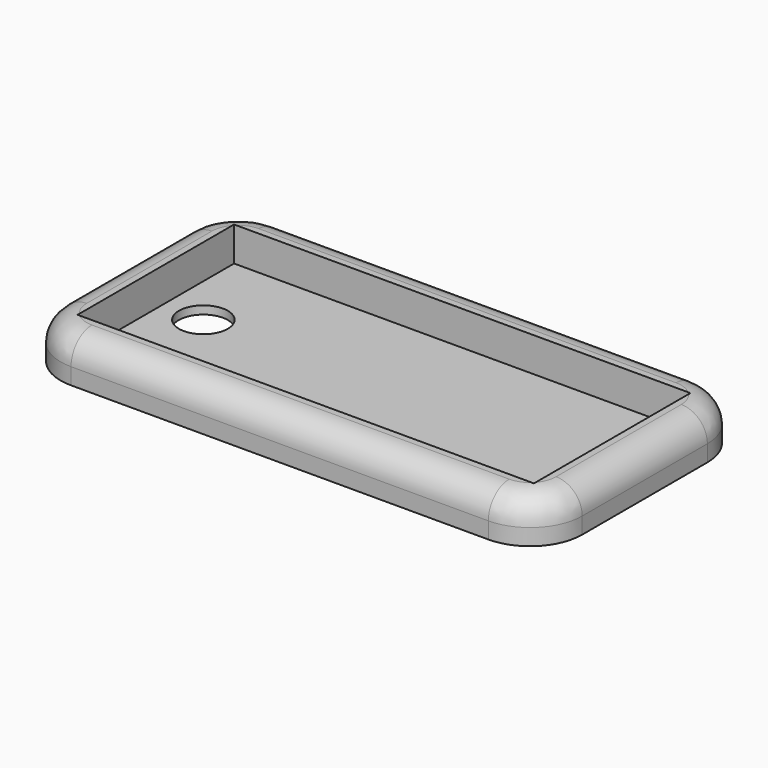
from build123d import *

# Parameters (mm, degrees)
F0_W         = 44.45
F0_H         = 19.05
F0_R         = 2.38125
F1_DEPTH     = 0.79375
F2_DEPTH     = 4.1402
F3_R         = 5.08
F4_T1_DEPTH  = 40.64
F4_T3_DEPTH  = 15.24
F4_T6_ANGLE  = 90
F4_T8_ANGLE  = 90
F4_T10_ANGLE = 90
F4_T12_ANGLE = 90


# Not quite as in the source:
# - a fillet or chamfer that OpenCascade refuses, or shapes differently, is made with other operations: its cross-section is extruded or revolved along the edge and cut away or added


with BuildPart() as f1:
    # F0 (on Top) → F1 (new body)
    with BuildSketch(Plane.XY):
        with Locations((25.4, 11.0452919405)):
            Rectangle(F0_W, F0_H)
        with Locations((7.14375, 11.8726459702)):
            Circle(F0_R, mode=Mode.SUBTRACT)
    extrude(amount=F1_DEPTH)

    # F0 (on Top) → F2 (join)
    with BuildSketch(Plane.XY):
        Polygon((0, 23.7452919405), (0, 0), (0, -1.6547080595), (50.8, -1.6547080595), (50.8, 23.7452919405), align=None)
        with Locations((25.4, 11.0452919405)):
            Rectangle(F0_W, F0_H, mode=Mode.SUBTRACT)
    extrude(amount=F2_DEPTH)

    # F3
    f3_edges = [f1.edges().sort_by_distance(p)[0] for p in [
        (50.8, -1.654708, 2.0701),
        (0, -1.654708, 2.0701),
        (50.8, 23.745292, 2.0701),
        (0, 23.745292, 2.0701),
    ]]
    fillet(f3_edges, radius=F3_R)

    # F4: fillet of radius 2.54 on 8 edges, made by hand

    # F4_s2 → F4_t1 (cut)
    with BuildSketch(Plane.YZ.offset(5.08)):
        with BuildLine():
            ThreePointArc((-1.6547080595, 1.6002), (-0.9107592837, 3.3962512242), (0.8852919405, 4.1402))
            Line((0.8852919405, 4.1402), (-1.6547080595, 4.1402))
            Line((-1.6547080595, 4.1402), (-1.6547080595, 1.6002))
        make_face()
        with BuildLine():
            ThreePointArc((23.7452919405, 1.6002), (23.0013431647, 3.3962512242), (21.2052919405, 4.1402))
            Line((21.2052919405, 4.1402), (23.7452919405, 4.1402))
            Line((23.7452919405, 4.1402), (23.7452919405, 1.6002))
        make_face()
    extrude(amount=F4_T1_DEPTH, mode=Mode.SUBTRACT)

    # F4_s4 → F4_t3 (cut)
    with BuildSketch(Plane.XZ.offset(-18.6652919405)):
        with BuildLine():
            ThreePointArc((0, 1.6002), (0.7439487758, 3.3962512242), (2.54, 4.1402))
            Line((2.54, 4.1402), (0, 4.1402))
            Line((0, 4.1402), (0, 1.6002))
        make_face()
        with BuildLine():
            ThreePointArc((50.8, 1.6002), (50.0560512242, 3.3962512242), (48.26, 4.1402))
            Line((48.26, 4.1402), (50.8, 4.1402))
            Line((50.8, 4.1402), (50.8, 1.6002))
        make_face()
    extrude(amount=F4_T3_DEPTH, mode=Mode.SUBTRACT)

    # F4_s5 → F4_t6 (revolve, cut)
    with BuildSketch(Plane.XZ.offset(-18.6652919405)):
        with BuildLine():
            ThreePointArc((0, 1.6002), (0.7439487758, 3.3962512242), (2.54, 4.1402))
            Line((2.54, 4.1402), (0, 4.1402))
            Line((0, 4.1402), (0, 1.6002))
        make_face()
    revolve(axis=Axis((5.08, 18.6652919405, 4.1402), (0, 0, -1)), revolution_arc=F4_T6_ANGLE, mode=Mode.SUBTRACT)

    # F4_s7 → F4_t8 (revolve, cut)
    with BuildSketch(Plane.XZ.offset(-3.4252919405)):
        with BuildLine():
            ThreePointArc((0, 1.6002), (0.7439487758, 3.3962512242), (2.54, 4.1402))
            Line((2.54, 4.1402), (0, 4.1402))
            Line((0, 4.1402), (0, 1.6002))
        make_face()
    revolve(axis=Axis((5.08, 3.4252919405, 4.1402), (0, 0, 1)), revolution_arc=F4_T8_ANGLE, mode=Mode.SUBTRACT)

    # F4_s9 → F4_t10 (revolve, cut)
    with BuildSketch(Plane.XZ.offset(-18.6652919405)):
        with BuildLine():
            ThreePointArc((50.8, 1.6002), (50.0560512242, 3.3962512242), (48.26, 4.1402))
            Line((48.26, 4.1402), (50.8, 4.1402))
            Line((50.8, 4.1402), (50.8, 1.6002))
        make_face()
    revolve(axis=Axis((45.72, 18.6652919405, 4.1402), (0, 0, 1)), revolution_arc=F4_T10_ANGLE, mode=Mode.SUBTRACT)

    # F4_s11 → F4_t12 (revolve, cut)
    with BuildSketch(Plane.YZ.offset(45.72)):
        with BuildLine():
            ThreePointArc((-1.6547080595, 1.6002), (-0.9107592837, 3.3962512242), (0.8852919405, 4.1402))
            Line((0.8852919405, 4.1402), (-1.6547080595, 4.1402))
            Line((-1.6547080595, 4.1402), (-1.6547080595, 1.6002))
        make_face()
    revolve(axis=Axis((45.72, 3.4252919405, 4.1402), (0, 0, 1)), revolution_arc=F4_T12_ANGLE, mode=Mode.SUBTRACT)


solid = f1.part
